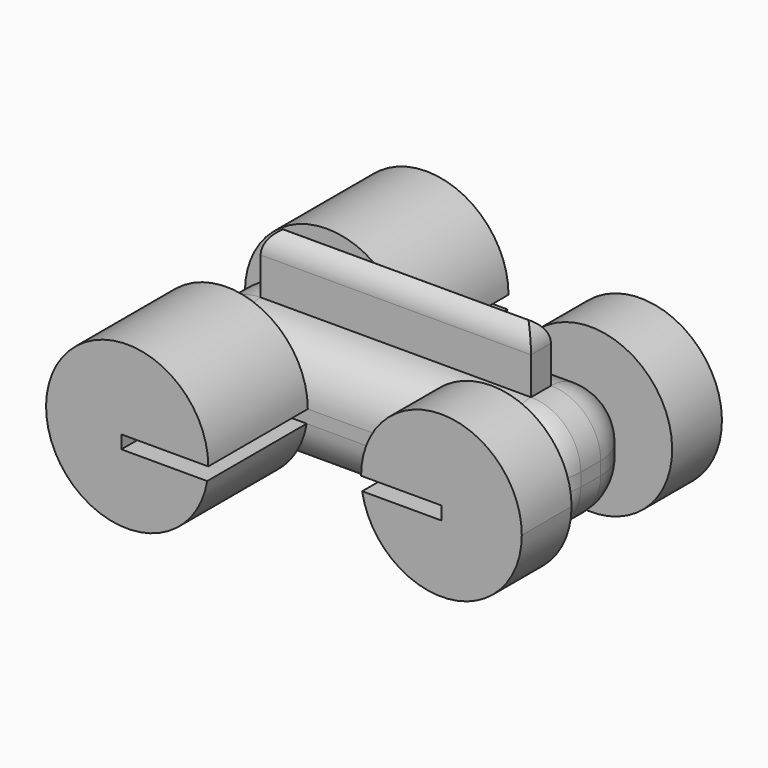
from build123d import *

# Parameters (mm, degrees)
F0_W         = 75.5182132125
F0_H         = 23.0204220861
F1_DEPTH     = 25.4
F2_R         = 10.16
F5_DEPTH     = 25.4
F6_DEPTH     = 25.4
F7_DEPTH     = 12.7
F8_DEPTH     = 12.7
F9_W         = 55.1982132125
F9_H         = 5.08
F10_DEPTH    = 12.7
F11_T1_DEPTH = 30.48
F11_T3_DEPTH = 80.5982132125


# Not quite as in the source:
# - a fillet or chamfer that OpenCascade refuses, or shapes differently, is made with other operations: its cross-section is extruded or revolved along the edge and cut away or added


with BuildPart() as f1:
    # F0 (on Front) → F1 (new body)
    with BuildSketch(Plane.XZ):
        with Locations((-37.7591066062, 11.5102110431)):
            Rectangle(F0_W, F0_H)
    extrude(amount=F1_DEPTH)

    # F2
    f2_edges = [f1.edges().sort_by_distance(p)[0] for p in [
        (-37.759107, -25.4, 0),
        (-75.518213, -12.7, 23.020422),
        (-75.518213, -12.7, 0),
        (-75.518213, 0, 11.510211),
        (-75.518213, -25.4, 11.510211),
        (-37.759107, 0, 0),
        (0, 0, 11.510211),
        (-37.759107, 0, 23.020422),
        (0, -12.7, 23.020422),
        (-37.759107, -25.4, 23.020422),
        (0, -12.7, 0),
        (0, -25.4, 11.510211),
    ]]
    fillet(f2_edges, radius=F2_R)

    # F9 (on face) → F10 (join)
    with BuildSketch(Plane.XY.offset(23.0204220861)):
        with Locations((-37.7591066062, -12.7)):
            Rectangle(F9_W, F9_H)
    extrude(amount=F10_DEPTH)

    # F11: fillet of radius 5.08 on 4 edges, made by hand

    # F11_s2 → F11_t1 (cut)
    with BuildSketch(Plane.XZ.offset(-2.54)):
        with BuildLine():
            ThreePointArc((-10.16, 30.6404220861), (-11.6478975516, 34.2325245345), (-15.24, 35.7204220861))
            Line((-15.24, 35.7204220861), (-10.16, 35.7204220861))
            Line((-10.16, 35.7204220861), (-10.16, 30.6404220861))
        make_face()
        with BuildLine():
            ThreePointArc((-65.3582132125, 30.6404220861), (-63.8703156609, 34.2325245345), (-60.2782132125, 35.7204220861))
            Line((-60.2782132125, 35.7204220861), (-65.3582132125, 35.7204220861))
            Line((-65.3582132125, 35.7204220861), (-65.3582132125, 30.6404220861))
        make_face()
    extrude(amount=F11_T1_DEPTH, mode=Mode.SUBTRACT)

    # F11_s4 → F11_t3 (cut)
    with BuildSketch(Plane.YZ.offset(-78.0582132125)):
        with BuildLine():
            ThreePointArc((-10.16, 30.6404220861), (-11.6478975516, 34.2325245345), (-15.24, 35.7204220861))
            Line((-15.24, 35.7204220861), (-10.16, 35.7204220861))
            Line((-10.16, 35.7204220861), (-10.16, 30.6404220861))
        make_face()
        with BuildLine():
            ThreePointArc((-15.24, 30.6404220861), (-13.7521024484, 34.2325245345), (-10.16, 35.7204220861))
            Line((-10.16, 35.7204220861), (-15.24, 35.7204220861))
            Line((-15.24, 35.7204220861), (-15.24, 30.6404220861))
        make_face()
    extrude(amount=F11_T3_DEPTH, mode=Mode.SUBTRACT)


with BuildPart() as f5:
    # F4 (on face) → F5 (new body)
    with BuildSketch(Plane.XZ.offset(25.4)):
        with BuildLine():
            Line((-65.3582132125, 12.8604220861), (-47.6042628759, 12.8604220861))
            ThreePointArc((-47.6042628759, 12.8604220861), (-80.6685369308, 14.2151742503), (-47.825925372, 10.16))
            Line((-47.825925372, 10.16), (-65.3582132125, 10.16))
            Line((-65.3582132125, 10.16), (-65.3582132125, 12.8604220861))
        make_face()
    extrude(amount=F5_DEPTH)


with BuildPart() as f6:
    # F3 (on face) → F6 (new body)
    with BuildSketch(Plane(origin=(0, 0, 0), x_dir=(-1, 0, 0), z_dir=(0, 1, 0))):
        with BuildLine():
            ThreePointArc((47.4824030652, 10.16), (65.3673252812, -3.83410232), (80.7620710494, 12.8604220861))
            ThreePointArc((80.7620710494, 12.8604220861), (64.0126764774, 29.6098166581), (47.2632819055, 12.8604220861))
            Line((47.2632819055, 12.8604220861), (65.3582132125, 12.8604220861))
            Line((65.3582132125, 12.8604220861), (65.3582132125, 10.16))
            Line((65.3582132125, 10.16), (47.4824030652, 10.16))
        make_face()
    extrude(amount=F6_DEPTH)


with BuildPart() as f7:
    # F4 (on face) → F7 (new body)
    with BuildSketch(Plane.XZ.offset(25.4)):
        with BuildLine():
            ThreePointArc((6.2484602862, 12.8604220861), (-10.16, 29.2688823724), (-26.5684602862, 12.8604220861))
            Line((-26.5684602862, 12.8604220861), (-10.16, 12.8604220861))
            Line((-10.16, 12.8604220861), (-10.16, 10.16))
            Line((-10.16, 10.16), (-26.3447239557, 10.16))
            ThreePointArc((-26.3447239557, 10.16), (-8.8051626123, -3.4920084555), (6.2484602862, 12.8604220861))
        make_face()
    extrude(amount=F7_DEPTH)


with BuildPart() as f8:
    # F3 (on face) → F8 (new body)
    with BuildSketch(Plane(origin=(0, 0, 0), x_dir=(-1, 0, 0), z_dir=(0, 1, 0))):
        with BuildLine():
            Line((10.16, 12.8604220861), (26.7926303068, 12.8604220861))
            ThreePointArc((26.7926303068, 12.8604220861), (-6.4173684927, 14.2151341519), (26.5719502644, 10.16))
            Line((26.5719502644, 10.16), (10.16, 10.16))
            Line((10.16, 10.16), (10.16, 12.8604220861))
        make_face()
    extrude(amount=F8_DEPTH)


solid = Compound([f1.part, f5.part, f6.part, f7.part, f8.part])
